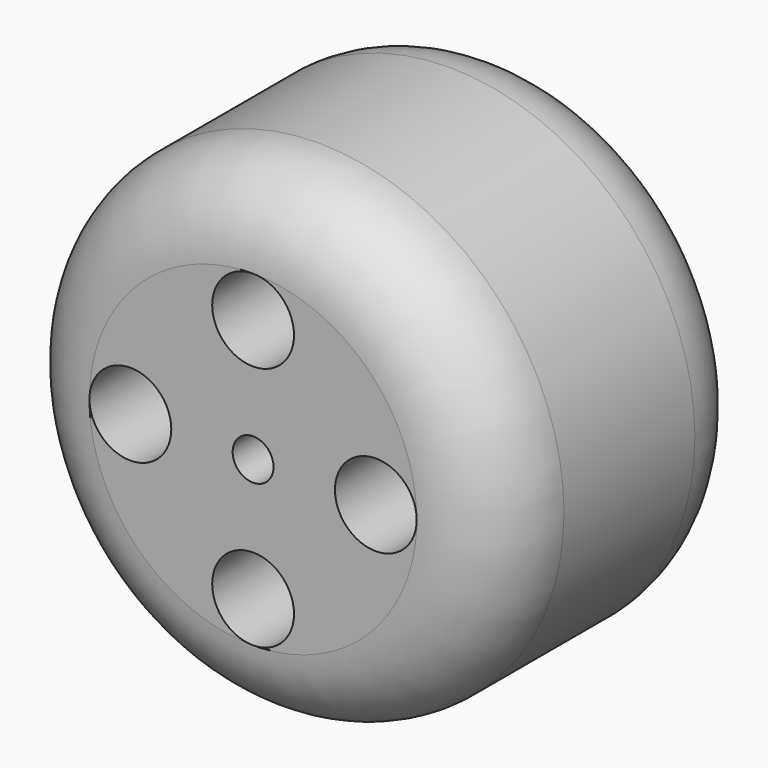
from build123d import *

# Parameters (mm, degrees)
F0_R     = 38.1
F0_R_2   = 6.35
F0_R_3   = 3.175
F1_DEPTH = 50.8
F2_R     = 12.69999
F3_R     = 12.69999


# Not quite as in the source:
# - a fillet or chamfer is up to 0.001 mm smaller than in the source, because OpenCascade refuses the exact size


with BuildPart() as f1:
    # F0 (on Front) → F1 (new body)
    with BuildSketch(Plane.XZ):
        Circle(F0_R)
        with Locations((0, -19.05)):
            Circle(F0_R_2, mode=Mode.SUBTRACT)
        with Locations((-19.05, 0)):
            Circle(F0_R_2, mode=Mode.SUBTRACT)
        Circle(F0_R_3, mode=Mode.SUBTRACT)
        with Locations((19.05, 0)):
            Circle(F0_R_2, mode=Mode.SUBTRACT)
        with Locations((0, 19.05)):
            Circle(F0_R_2, mode=Mode.SUBTRACT)
    extrude(amount=F1_DEPTH)

    # F2 (radius 12.7 in the source; OpenCascade refuses exactly that, so slightly less here)
    f2_edges = [f1.edges().sort_by_distance(p)[0] for p in [
        (-38.1, -50.8, 0),
    ]]
    fillet(f2_edges, radius=F2_R)

    # F3 (radius 12.7 in the source; OpenCascade refuses exactly that, so slightly less here)
    f3_edges = [f1.edges().sort_by_distance(p)[0] for p in [
        (-38.1, 0, 0),
    ]]
    fillet(f3_edges, radius=F3_R)


solid = f1.part
